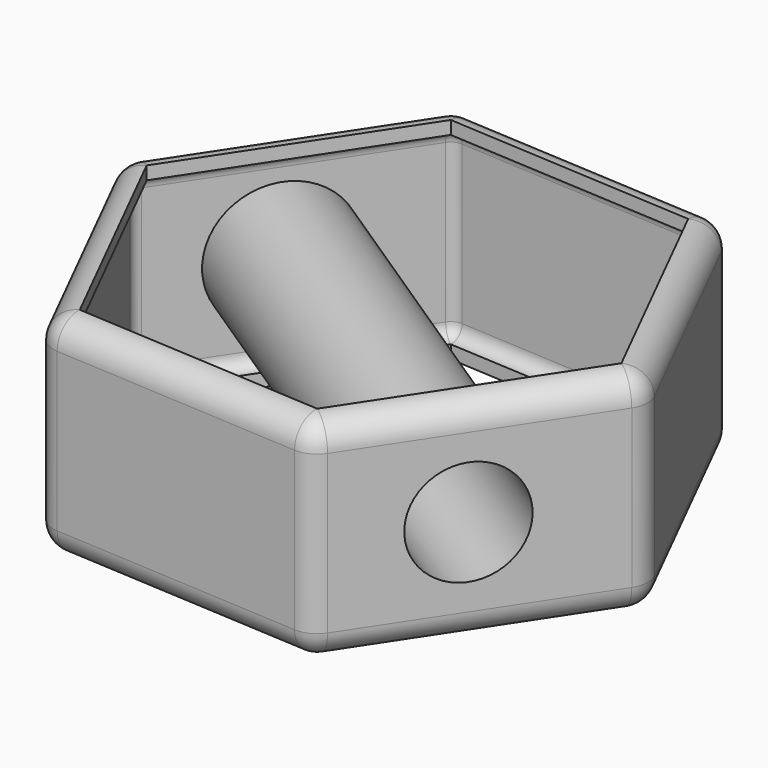
from build123d import *

# Parameters (mm, degrees)
F1_DEPTH       = 40
F2_R           = 5
F4_D           = 20
F4_CBORE_D     = 20
F4_CBORE_DEPTH = 20
F5_T           = -2.5


# Not quite as in the source:
# - a shell that OpenCascade refuses in one call is made with other operations: the cavity is built on its own and cut out


with BuildPart() as f1:
    # F0 (on Top) → F1 (new body)
    with BuildSketch(Plane.XY):
        Polygon((29.2738805136, 44.3878389125), (-23.8040558605, 47.5458436484), (-53.0779363741, 3.1580047359), (-29.2738805136, -44.3878389125), (23.8040558605, -47.5458436484), (53.0779363741, -3.1580047359), align=None)
    extrude(amount=F1_DEPTH)

    # F2
    f2_edges = [f1.edges().sort_by_distance(p)[0] for p in [
        (2.734912, 45.966841, 40),
        (41.175908, 20.614917, 40),
        (38.440996, -25.351924, 40),
        (-2.734912, -45.966841, 40),
        (-41.175908, -20.614917, 40),
        (-38.440996, 25.351924, 40),
        (29.273881, 44.387839, 20),
        (-23.804056, 47.545844, 20),
        (-53.077936, 3.158005, 20),
        (-29.273881, -44.387839, 20),
        (23.804056, -47.545844, 20),
        (53.077936, -3.158005, 20),
        (41.175908, 20.614917, 0),
        (38.440996, -25.351924, 0),
        (-2.734912, -45.966841, 0),
        (-41.175908, -20.614917, 0),
        (-38.440996, 25.351924, 0),
        (2.734912, 45.966841, 0),
    ]]
    fillet(f2_edges, radius=F2_R)

    # F4 (through all)
    with Locations(Plane(origin=(-38.4409961173, 25.3519241922, 0), x_dir=(-0.5505527454, -0.83480038, 0), z_dir=(-0.83480038, 0.5505527454, 0))):
        with Locations((1.7491957406, 20)):
            CounterBoreHole(F4_D / 2, F4_CBORE_D / 2, F4_CBORE_DEPTH)

    # F5: a shell. OpenCascade refuses it in one call, so the cavity is built on its own and cut out:
    # the body offset inwards by the wall thickness, plus a prism from it out through each open face.
    f5_core = offset(f1.part, amount=F5_T, mode=Mode.PRIVATE)
    f5_exits = [f5_core.faces().sort_by_distance(p)[0] for p in [
        (0, 0, 2.5),
        (0, 0, 37.5),
    ]]
    add(f5_core, mode=Mode.SUBTRACT)
    extrude(f5_exits, amount=-F5_T, mode=Mode.SUBTRACT)


solid = f1.part
